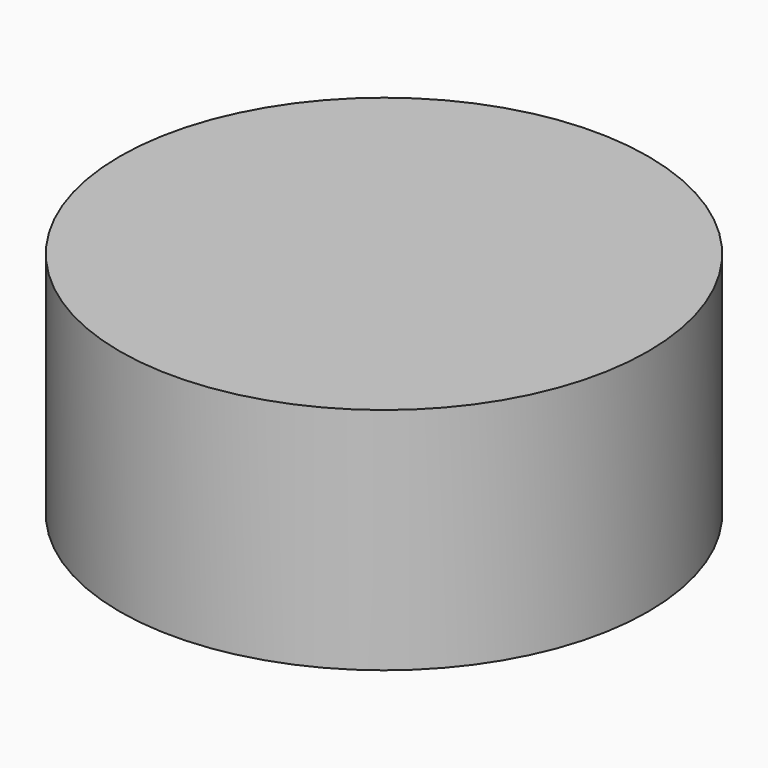
from build123d import *

# Parameters (mm, degrees)
F1_R     = 69.1587452347
F2_DEPTH = 60
F3_R     = 69.1587452347
F3_R_2   = 35.7120494857
F4_DEPTH = 25


# Not quite as in the source:
# - the program builds the solid bodies; features that only make, move or delete a surface that nothing else refers to are left out


with BuildPart() as f2:
    # F1 (on face) → F2 (new body)
    with BuildSketch(Plane.XY):
        Circle(F1_R)
    extrude(amount=F2_DEPTH)

    # F3 (on face) → F4 (join)
    with BuildSketch(Plane.XY):
        Circle(F3_R)
        Circle(F3_R_2, mode=Mode.SUBTRACT)
    extrude(amount=F4_DEPTH)


solid = f2.part
